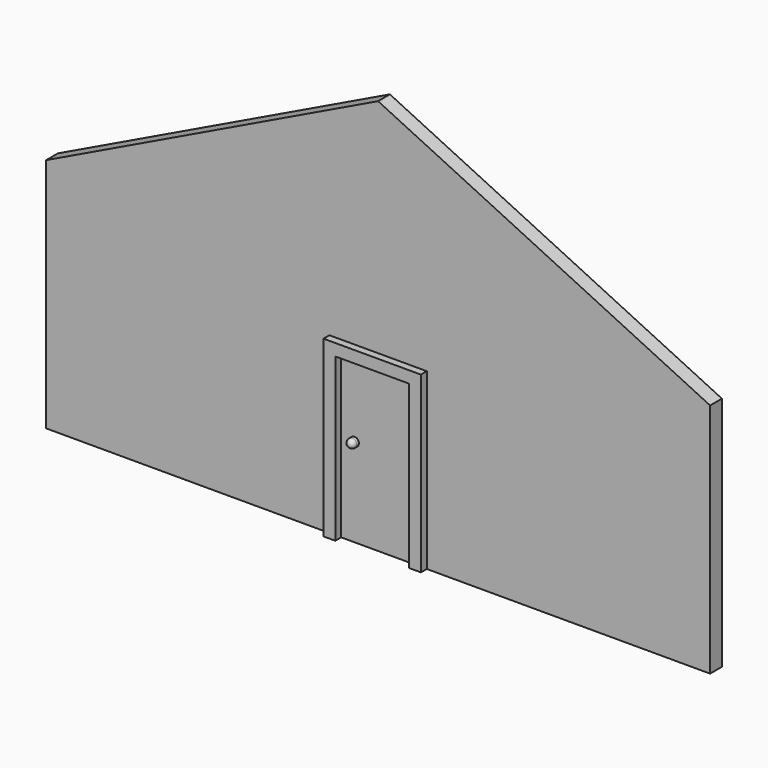
from build123d import *

# Parameters (mm, degrees)
F1_DEPTH = 2.54
F0_W     = 12.7
F0_H     = 27.94
F0_R     = 0.762
F2_DEPTH = 3.81
F3_DEPTH = 3.81
F4_R     = 0.762


# Not quite as in the source:
# - a feature names something its author has since deleted; it is built from what else it names


with BuildPart() as f1:
    # F0 (on Front) → F1 (new body)
    with BuildSketch(Plane.XZ):
        Polygon((0, 54.1968159378), (-57.15, 26.67), (57.15, 26.67), align=None)
        Polygon((-57.15, -13.97), (-8.382, -13.97), (-8.382, 16.002), (8.382, 16.002), (8.382, -13.97), (57.15, -13.97), (57.15, 26.67), (-57.15, 26.67), align=None)
    extrude(amount=F1_DEPTH)



with BuildPart() as f1b:
    # F0 (on Front) → F1, piece 2 (new body)
    with BuildSketch(Plane.XZ):
        Rectangle(F0_W, F0_H)
        with Locations((-4.064, 1.27)):
            Circle(F0_R, mode=Mode.SUBTRACT)
    extrude(amount=F1_DEPTH)


with BuildPart() as f1_1:
    add(f1.part)

    add(f1b.part)  # F2 merges F1b
    # F0 (on Front) → F2 (join)
    with BuildSketch(Plane.XZ):
        Polygon((-6.35, -13.97), (-6.35, 13.97), (6.35, 13.97), (6.35, -13.97), (8.382, -13.97), (8.382, 16.002), (-8.382, 16.002), (-8.382, -13.97), align=None)
    extrude(amount=F2_DEPTH)

    # F0 (on Front) → F3 (join)
    with BuildSketch(Plane.XZ):
        with Locations((-4.064, 1.27)):
            Circle(F0_R)
    extrude(amount=F3_DEPTH)

    # F4
    f4_edges = [f1_1.edges().sort_by_distance(p)[0] for p in [
        (-4.826, -3.81, 1.27),
    ]]
    fillet(f4_edges, radius=F4_R)


solid = f1_1.part
